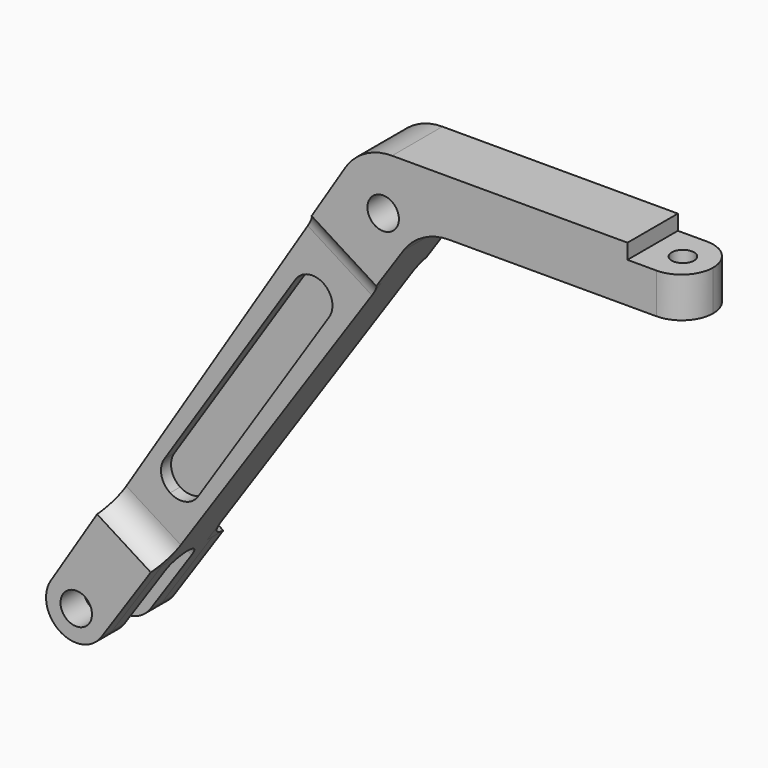
from build123d import *

# Parameters (mm, degrees)
F0_R          = 1.5875
F1_DEPTH      = 6.35
F3_D          = 2.2606
F4_R          = 3.17499
F5_R          = 1.5875
F6_DEPTH      = 1.397
F7_R          = 1.5875
F8_DEPTH      = 1.397
F10_DEPTH     = 55.922402023
F11_W         = 0.635
F11_H         = 38.4961159321
F12_DEPTH     = 55.922402023
F13_T4_DEPTH  = 12.6181992369
F13_T9_DEPTH  = 12.6181992369
F13_T14_DEPTH = 11.9054737587
F13_T19_DEPTH = 11.9054737587
F15_DEPTH     = 1.27
F17_DEPTH     = 1.27


# Not quite as in the source:
# - a fillet or chamfer that OpenCascade refuses, or shapes differently, is made with other operations: its cross-section is extruded or revolved along the edge and cut away or added
# - a fillet or chamfer is up to 0.001 mm smaller than in the source, because OpenCascade refuses the exact size


with BuildPart() as f1:
    # F0 (on Front) → F1 (new body)
    with BuildSketch(Plane.XZ):
        with BuildLine():
            Line((6.6774413169, -0.1881909028), (30.734, -0.1881909028))
            Line((30.734, -0.1881909028), (30.734, 3.8758090972))
            Line((30.734, 3.8758090972), (24.638, 3.8758090972))
            Line((24.638, 3.8758090972), (24.638, 5.3998090972))
            Line((24.638, 5.3998090972), (0.8976435847, 5.3998090972))
            ThreePointArc((0.8976435847, 5.3998090972), (-1.8031521678, 4.7037868469), (-3.8311440773, 2.7891084184))
            Line((-3.8311440773, 2.7891084184), (-32.4066881959, -42.5968826722))
            ThreePointArc((-32.4066881959, -42.5968826722), (-31.4949255527, -46.7722351265), (-27.3046829217, -45.931553303))
            Line((-27.3046829217, -45.931553303), (2.052552643, -2.6399274008))
            ThreePointArc((2.052552643, -2.6399274008), (4.0601618562, -0.8390265117), (6.6774413169, -0.1881909028))
        make_face()
        with Locations((-29.8273494711, -44.2208641201)):
            Circle(F0_R, mode=Mode.SUBTRACT)
        Circle(F0_R, mode=Mode.SUBTRACT)
    extrude(amount=F1_DEPTH)

    # F3 (through all)
    with Locations(Plane.XY.offset(3.8758090972)):
        with Locations((27.686, -3.175)):
            Hole(F3_D / 2)

    # F4 (radius 3.175 in the source; OpenCascade refuses exactly that, so slightly less here)
    f4_edges = [f1.edges().sort_by_distance(p)[0] for p in [
        (30.734, -6.35, 1.843809),
        (30.734, 0, 1.843809),
    ]]
    fillet(f4_edges, radius=F4_R)

    # F5 (on face) → F6 (join)
    with BuildSketch(Plane.XZ.offset(6.35)):
        with BuildLine():
            Line((-27.3046829217, -45.931553303), (-22.3122897877, -38.5695244281))
            Line((-22.3122897877, -38.5695244281), (-27.7252582931, -35.1614569468))
            Line((-27.7252582931, -35.1614569468), (-32.4066881959, -42.5968826722))
            ThreePointArc((-32.4066881959, -42.5968826722), (-31.4949255527, -46.7722351265), (-27.3046829217, -45.931553303))
        make_face()
        with Locations((-29.8273494711, -44.2208641201)):
            Circle(F5_R, mode=Mode.SUBTRACT)
    extrude(amount=F6_DEPTH)

    # F7 (on face) → F8 (join)
    with BuildSketch(Plane(origin=(0, 0, 0), x_dir=(-1, 0, 0), z_dir=(0, 1, 0))):
        with BuildLine():
            ThreePointArc((27.3046829217, -45.931553303), (31.4949255527, -46.7722351265), (32.4066881959, -42.5968826722))
            Line((32.4066881959, -42.5968826722), (27.7252582931, -35.1614569468))
            Line((27.7252582931, -35.1614569468), (22.3122897877, -38.5695244281))
            Line((22.3122897877, -38.5695244281), (27.3046829217, -45.931553303))
        make_face()
        with Locations((29.8273494711, -44.2208641201)):
            Circle(F7_R, mode=Mode.SUBTRACT)
    extrude(amount=F8_DEPTH)

    # F9 (on face) → F10 (cut, through all)
    with BuildSketch(Plane(origin=(-4.0011143857, 0, 2.519147823), x_dir=(0, -1, 0), z_dir=(-0.8462397391, 0, 0.5328023123))):
        with BuildLine():
            Line((1.524, -56.3615332831), (4.826, -56.3615332831))
            Line((4.826, -56.3615332831), (4.826, -46.0745332831))
            ThreePointArc((4.826, -46.0745332831), (3.175, -44.4235332831), (1.524, -46.0745332831))
            Line((1.524, -46.0745332831), (1.524, -56.3615332831))
        make_face()
    extrude(amount=-F10_DEPTH, mode=Mode.SUBTRACT)

    # F11 (on face) → F12 (cut, through all)
    with BuildSketch(Plane(origin=(-4.0011143857, 0, 2.519147823), x_dir=(0, -1, 0), z_dir=(-0.8462397391, 0, 0.5328023123))):
        with Locations((0.3175, -25.2790459142)):
            Rectangle(F11_W, F11_H)
        with Locations((6.0325, -25.2790459142)):
            Rectangle(F11_W, F11_H)
    extrude(amount=-F12_DEPTH, mode=Mode.SUBTRACT)

    # F13: fillet of radius 2.54 on 4 edges, made by hand


with BuildPart() as f13_tool2:
    # F13_s3 → F13_t4 (new body)
    with BuildSketch(Plane(origin=(-4.0011143857, 0, 2.519147823), x_dir=(0, 1, 0), z_dir=(0.8462397391, 0, -0.5328023123))):
        with BuildLine():
            ThreePointArc((-7.747, -44.5271038802), (-6.2875244601, -43.6448593529), (-5.715, -42.0384223016))
            Line((-5.715, -42.0384223016), (-5.715, -44.5271038802))
            Line((-5.715, -44.5271038802), (-7.747, -44.5271038802))
        make_face()
    extrude(amount=F13_T4_DEPTH)

    split(bisect_by=Plane(origin=(2.6322854892, 0, -1.7850247841), x_dir=(0, 1, 0), z_dir=(-0.8276465057, 0, 0.5612497319)), keep=Keep.TOP)


with BuildPart() as f1_1:
    add(f1.part)

    # F13_t1: union F13_tool2
    add(f13_tool2.part)


with BuildPart() as f13_tool7:
    # F13_s8 → F13_t9 (new body)
    with BuildSketch(Plane(origin=(-4.0011143857, 0, 2.519147823), x_dir=(0, 1, 0), z_dir=(0.8462397391, 0, -0.5328023123))):
        with BuildLine():
            ThreePointArc((-0.635, -42.0384223016), (-0.0624755399, -43.6448593529), (1.397, -44.5271038802))
            Line((1.397, -44.5271038802), (-0.635, -44.5271038802))
            Line((-0.635, -44.5271038802), (-0.635, -42.0384223016))
        make_face()
    extrude(amount=F13_T9_DEPTH)

    split(bisect_by=Plane(origin=(2.6322854892, 0, -1.7850247841), x_dir=(0, 1, 0), z_dir=(-0.8276465057, 0, 0.5612497319)), keep=Keep.TOP)


with BuildPart() as f1_2:
    add(f1_1.part)

    # F13_t6: union F13_tool7
    add(f13_tool7.part)


with BuildPart() as f13_tool12:
    # F13_s13 → F13_t14 (new body)
    with BuildSketch(Plane(origin=(-4.0011143857, 0, 2.519147823), x_dir=(0, 1, 0), z_dir=(0.8462397391, 0, -0.5328023123))):
        with BuildLine():
            ThreePointArc((0, -6.0309879482), (-0.4709524406, -6.8130144186), (-0.635, -7.7110400307))
            Line((-0.635, -7.7110400307), (-0.635, -6.0309879482))
            Line((-0.635, -6.0309879482), (0, -6.0309879482))
        make_face()
    extrude(amount=F13_T14_DEPTH)

    split(bisect_by=Plane(origin=(2.6322854892, 0, -1.7850247841), x_dir=(0, 1, 0), z_dir=(-0.8276465057, 0, 0.5612497319)), keep=Keep.TOP)


with BuildPart() as f1_3:
    add(f1_2.part)

    # F13_t11: union F13_tool12
    add(f13_tool12.part)


with BuildPart() as f13_tool17:
    # F13_s18 → F13_t19 (new body)
    with BuildSketch(Plane(origin=(-4.0011143857, 0, 2.519147823), x_dir=(0, 1, 0), z_dir=(0.8462397391, 0, -0.5328023123))):
        with BuildLine():
            ThreePointArc((-5.715, -7.7110400307), (-5.8790475594, -6.8130144186), (-6.35, -6.0309879482))
            Line((-6.35, -6.0309879482), (-5.715, -6.0309879482))
            Line((-5.715, -6.0309879482), (-5.715, -7.7110400307))
        make_face()
    extrude(amount=F13_T19_DEPTH)

    split(bisect_by=Plane(origin=(2.6322854892, 0, -1.7850247841), x_dir=(0, 1, 0), z_dir=(-0.8276465057, 0, 0.5612497319)), keep=Keep.TOP)


with BuildPart() as f1_4:
    add(f1_3.part)

    # F13_t16: union F13_tool17
    add(f13_tool17.part)

    # F14 (on face) → F15 (cut)
    with BuildSketch(Plane.XZ.offset(5.715)):
        with BuildLine():
            ThreePointArc((-22.5785911234, -29.4180135738), (-22.8665153513, -30.9463544712), (-21.9894083128, -32.2306478578))
            ThreePointArc((-21.9894083128, -32.2306478578), (-20.4610674153, -32.5185720857), (-19.1767740287, -31.6414650472))
            Line((-19.1767740287, -31.6414650472), (-5.9518651728, -11.4077331396))
            ThreePointArc((-5.9518651728, -11.4077331396), (-5.6639409449, -9.8793922421), (-6.5410479835, -8.5950988555))
            ThreePointArc((-6.5410479835, -8.5950988555), (-8.0693888809, -8.3071746276), (-9.3536822675, -9.1842816662))
            Line((-9.3536822675, -9.1842816662), (-22.5785911234, -29.4180135738))
        make_face()
    extrude(amount=-F15_DEPTH, mode=Mode.SUBTRACT)

    # F16 (on face) → F17 (cut)
    with BuildSketch(Plane(origin=(0, -0.635, 0), x_dir=(-1, 0, 0), z_dir=(0, 1, 0))):
        with BuildLine():
            ThreePointArc((19.1767740287, -31.6414650472), (21.9894083128, -32.2306478578), (22.5785911234, -29.4180135738))
            Line((22.5785911234, -29.4180135738), (9.3536822675, -9.1842816662))
            ThreePointArc((9.3536822675, -9.1842816662), (6.5410479835, -8.5950988555), (5.9518651728, -11.4077331396))
            Line((5.9518651728, -11.4077331396), (19.1767740287, -31.6414650472))
        make_face()
    extrude(amount=-F17_DEPTH, mode=Mode.SUBTRACT)


solid = f1_4.part
